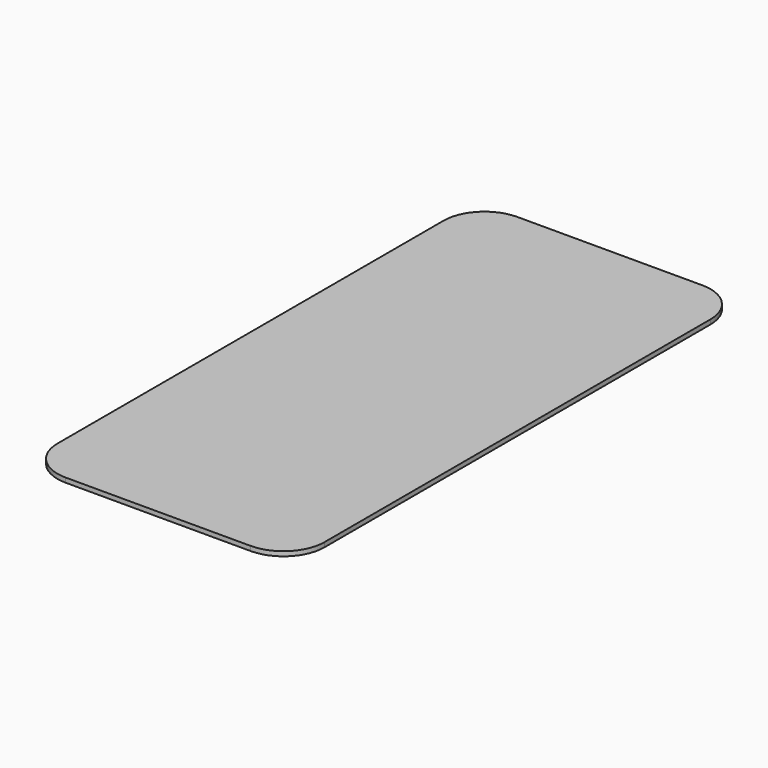
from build123d import *

# Parameters (mm, degrees)
F1_DEPTH = 1


# Not quite as in the source:
# - a feature of the source that left no trace in its solid (it failed there, or was rolled back) is left out


with BuildPart() as f1:
    # F0 (on Top) → F1 (new body)
    with BuildSketch(Plane.XY):
        with BuildLine():
            ThreePointArc((29.285, 52.915), (26.6489610307, 59.2789610307), (20.285, 61.915))
            Line((20.285, 61.915), (-20.285, 61.915))
            ThreePointArc((-20.285, 61.915), (-26.6489610307, 59.2789610307), (-29.285, 52.915))
            Line((-29.285, 52.915), (-29.285, -52.915))
            ThreePointArc((-29.285, -52.915), (-26.6489610307, -59.2789610307), (-20.285, -61.915))
            Line((-20.285, -61.915), (20.285, -61.915))
            ThreePointArc((20.285, -61.915), (26.6489610307, -59.2789610307), (29.285, -52.915))
            Line((29.285, -52.915), (29.285, 52.915))
        make_face()
    extrude(amount=F1_DEPTH)


solid = f1.part
